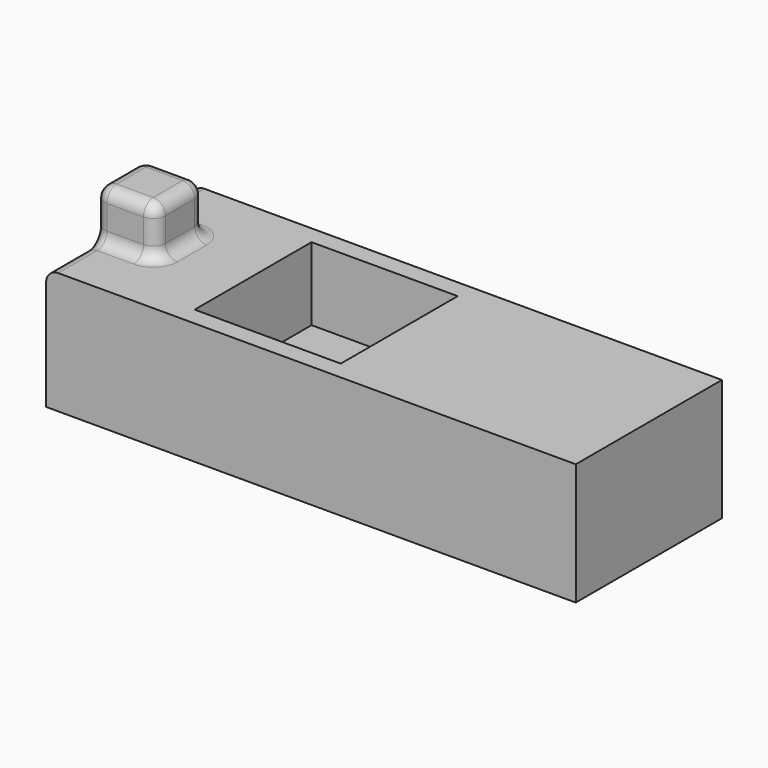
from build123d import *

# Parameters (mm, degrees)
F0_W     = 47.625
F0_H     = 19.05
F1_DEPTH = 12.7
F3_DEPTH = 7.62
F4_W     = 19.05
F4_H     = 12.7
F5_DEPTH = 7.62
F7_DEPTH = 5.08
F8_R     = 1.27


with BuildPart() as f1:
    # F0 (on Top) → F1 (new body)
    with BuildSketch(Plane.XY):
        Rectangle(F0_W, F0_H)
    extrude(amount=F1_DEPTH)

    # F2 (on face) → F3 (cut)
    with BuildSketch(Plane.XY.offset(12.7)):
        Polygon((-17.4625, -7.62), (-2.2225, -7.62), (-2.2225, 0), (-2.2225, 7.62), (-17.4625, 7.62), align=None)
    extrude(amount=-F3_DEPTH, mode=Mode.SUBTRACT)

    # F4 (on face) → F5 (join)
    with BuildSketch(Plane(origin=(-23.8125, 0, 0), x_dir=(0, -1, 0), z_dir=(-1, 0, 0))):
        with Locations((0, 6.35)):
            Rectangle(F4_W, F4_H)
    extrude(amount=F5_DEPTH)

    # F6 (on face) → F7 (join)
    with BuildSketch(Plane.XY.offset(12.7)):
        Polygon((-28.2575, 3.175), (-31.4325, 3.175), (-31.4325, -3.175), (-25.0825, -3.175), (-25.0825, 3.175), align=None)
    extrude(amount=F7_DEPTH)

    # F8
    f8_edges = [f1.edges().sort_by_distance(p)[0] for p in [
        (-31.4325, 0, 17.78),
        (-25.0825, 0, 17.78),
        (-25.0825, -3.175, 15.24),
        (-28.2575, -3.175, 17.78),
        (-28.2575, 3.175, 17.78),
        (-31.4325, -3.175, 15.24),
        (-28.2575, -3.175, 12.7),
        (-25.0825, 0, 12.7),
        (-28.2575, 3.175, 12.7),
        (-31.4325, 3.175, 15.24),
        (-25.0825, 3.175, 15.24),
        (-31.4325, -6.35, 12.7),
        (-31.4325, 6.35, 12.7),
    ]]
    fillet(f8_edges, radius=F8_R)


solid = f1.part
